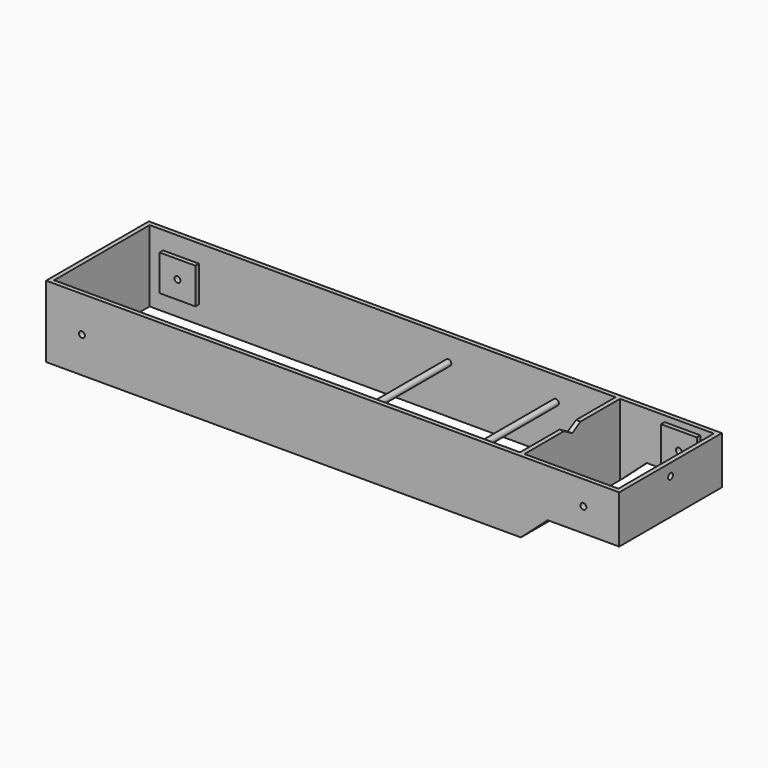
from build123d import *

# Parameters (mm, degrees)
F0_R      = 3.175
F1_DEPTH  = 4.7625
F2_W      = 4.7625
F2_H      = 50.8
F2_H_2    = 76.2
F2_R      = 3.175
F3_DEPTH  = 127
F4_R      = 3.175
F5_DEPTH  = 4.7625
F6_R      = 3.175
F7_DEPTH  = 25.4
F9_DEPTH  = 25.4
F10_W     = 38.1
F10_H     = 38.1
F10_R     = 3.175
F11_DEPTH = 4.7625
F12_W     = 38.1
F12_H     = 38.1
F12_R     = 3.175
F13_DEPTH = 4.7625
F14_W     = 38.1
F14_H     = 38.1
F14_R     = 3.175
F15_DEPTH = 4.7625
F16_W     = 38.1
F16_H     = 38.1
F16_R     = 3.175
F17_DEPTH = 4.7625


# Not quite as in the source:
# - a length typed as a fraction of an inch, garbled in the dataset ("3 / 203.2 mm" for 3/8 in), is restored


with BuildPart() as f1:
    # F0 (on Front) → F1 (new body)
    with BuildSketch(Plane.XZ):
        Polygon((0, 76.2), (0, 0), (505.0019366858, 0), (533.4, 25.4), (609.6, 25.4), (609.6, 76.2), align=None)
        with Locations((38.1, 38.1)):
            Circle(F0_R, mode=Mode.SUBTRACT)
        with Locations((571.5, 50.8)):
            Circle(F0_R, mode=Mode.SUBTRACT)
    extrude(amount=F1_DEPTH)

    # F2 (on face) → F3 (join)
    with BuildSketch(Plane(origin=(0, 0, 0), x_dir=(-1, 0, 0), z_dir=(0, 1, 0))):
        with Locations((-607.21875, 50.8)):
            Rectangle(F2_W, F2_H)
        with Locations((-502.6206866858, 38.1)):
            Rectangle(F2_W, F2_H_2)
        with Locations((-436.7394366858, 50.8)):
            Circle(F2_R)
        with Locations((-322.4394366858, 50.8)):
            Circle(F2_R)
        with Locations((-2.38125, 38.1)):
            Rectangle(F2_W, F2_H_2)
    extrude(amount=F3_DEPTH)

    # F4 (on face) → F5 (join)
    with BuildSketch(Plane(origin=(0, 127, 0), x_dir=(-1, 0, 0), z_dir=(0, 1, 0))):
        Polygon((0, 76.2), (-609.6, 76.2), (-609.6, 25.4), (-533.4, 25.4), (-505.0019366858, 0), (0, 0), align=None)
        with Locations((-571.5, 50.8)):
            Circle(F4_R, mode=Mode.SUBTRACT)
        with Locations((-38.1, 38.1)):
            Circle(F4_R, mode=Mode.SUBTRACT)
    extrude(amount=F5_DEPTH)

    # F6 (on face) → F7 (cut)
    with BuildSketch(Plane.YZ.offset(609.6)):
        with Locations((63.5, 63.5)):
            Circle(F6_R)
    extrude(amount=-F7_DEPTH, mode=Mode.SUBTRACT)

    # F8 (on face) → F9 (cut)
    with BuildSketch(Plane.YZ.offset(505.0019366858)):
        Polygon((74.4985226281, 76.2), (63.5, 76.2), (63.5, 69.85), align=None)
        Polygon((63.5, 69.85), (63.5, 76.2), (52.5014773719, 76.2), align=None)
    extrude(amount=-F9_DEPTH, mode=Mode.SUBTRACT)

    # F10 (on face) → F11 (join)
    with BuildSketch(Plane(origin=(0, 0, 0), x_dir=(-1, 0, 0), z_dir=(0, 1, 0))):
        with Locations((-38.1, 38.1)):
            Rectangle(F10_W, F10_H)
        with Locations((-38.1, 38.1)):
            Circle(F10_R, mode=Mode.SUBTRACT)
    extrude(amount=F11_DEPTH)

    # F12 (on face) → F13 (join)
    with BuildSketch(Plane(origin=(0, 0, 0), x_dir=(-1, 0, 0), z_dir=(0, 1, 0))):
        with Locations((-571.5, 50.8)):
            Rectangle(F12_W, F12_H)
        with Locations((-571.5, 50.8)):
            Circle(F12_R, mode=Mode.SUBTRACT)
    extrude(amount=F13_DEPTH)

    # F14 (on face) → F15 (join)
    with BuildSketch(Plane(origin=(0, 127, 0), x_dir=(-1, 0, 0), z_dir=(0, 1, 0))):
        with Locations((-38.1, 38.1)):
            Rectangle(F14_W, F14_H)
        with Locations((-38.1, 38.1)):
            Circle(F14_R, mode=Mode.SUBTRACT)
    extrude(amount=-F15_DEPTH)

    # F16 (on face) → F17 (join)
    with BuildSketch(Plane(origin=(0, 127, 0), x_dir=(-1, 0, 0), z_dir=(0, 1, 0))):
        with Locations((-571.5, 50.8)):
            Rectangle(F16_W, F16_H)
        with Locations((-571.5, 50.8)):
            Circle(F16_R, mode=Mode.SUBTRACT)
    extrude(amount=-F17_DEPTH)


solid = f1.part
